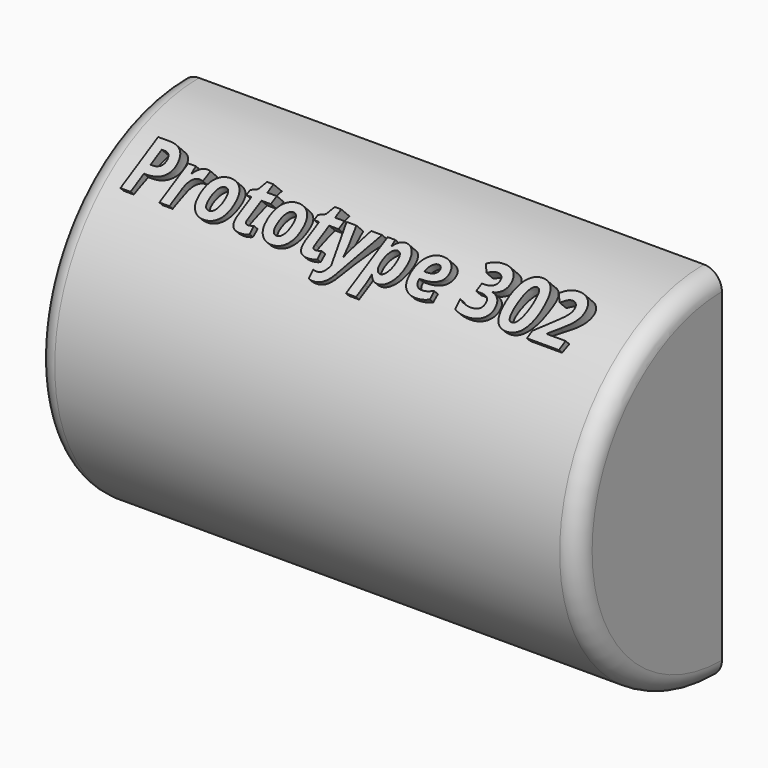
from build123d import *

# Parameters (mm, degrees)
F0_W         = 30
F0_H         = 10
F1_ANGLE     = 180
F2_T         = -1.5
F3_R         = 1
F6_TEXT_SIZE = 3.7734959081


# Not quite as in the source:
# - Text() gives the source's letters only with a copy of the font that has no kerning and outlines rounded to 1/6400 em; it was checked with that copy


with BuildPart() as f1:
    # F0 (on Front) → F1 (revolve)
    with BuildSketch(Plane.XZ):
        with Locations((15, 5)):
            Rectangle(F0_W, F0_H)
    revolve(axis=Axis((15, 0, 0), (1, 0, 0)), revolution_arc=F1_ANGLE)

    # F2
    f2_openings = [f1.faces().sort_by_distance(p)[0] for p in [
        (15, 0, 0),
    ]]
    offset(amount=F2_T, openings=f2_openings)

    # F3
    f3_edges = [f1.edges().sort_by_distance(p)[0] for p in [
        (0, -10, 0),
        (30, -10, 0),
    ]]
    fillet(f3_edges, radius=F3_R)

    # F6 (on face) → F7 (join, up to the next surface of F1)
    with BuildSketch(Plane(origin=(0, -7.2831998462, 7.2831998462), x_dir=(1, 0, 0), z_dir=(0, -0.7071067812, 0.7071067812))):
        with Locations((2, 0.6579892783)):
            Text('Prototype 302', F6_TEXT_SIZE, font='Open Sans', font_style=FontStyle.BOLDITALIC, text_align=(TextAlign.LEFT, TextAlign.BOTTOM))
    extrude(until=Until.NEXT, dir=(0, 0.7071067812, -0.7071067812))


solid = f1.part
